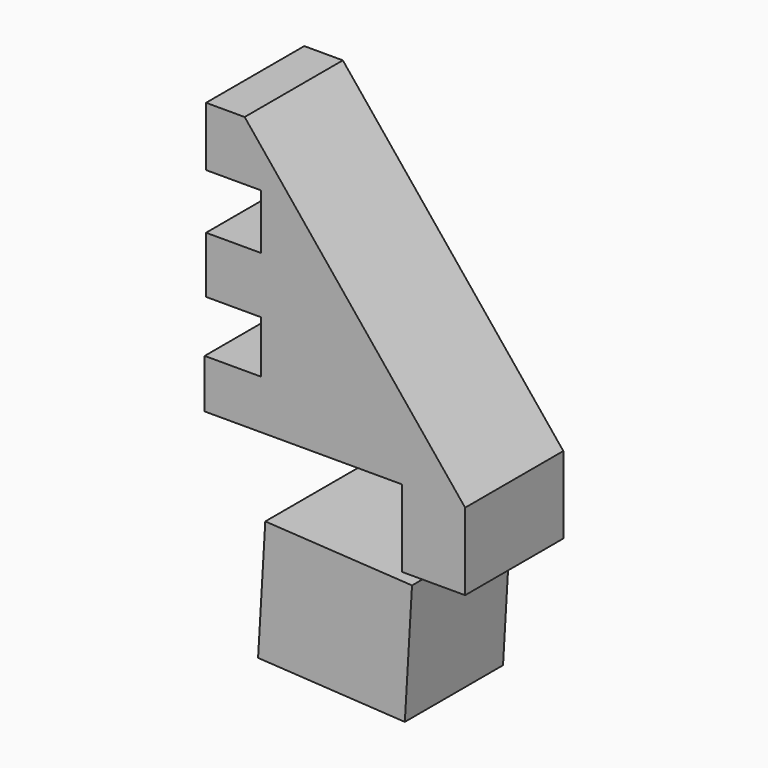
from build123d import *

# Parameters (mm, degrees)
F0_W     = 13.1069884534
F0_H     = 15.9477586227
F2_DEPTH = 25.4
F1_E23_W = 30.420306172
F1_E23_H = 25.4
F3_DEPTH = 25.4


with BuildPart() as f2:
    # F0 (on Front) → F2 (new body)
    with BuildSketch(Plane.XZ):
        Polygon((-3.4228879958, 56.3350282609), (-11.4096244797, 56.3350282609), (-11.4096244797, 44.0696775913), (0, 44.0696775913), (0, 32.6600521803), (-11.4096244797, 32.6600521803), (-11.4096244797, 20.9651887417), (0, 20.9651887417), (0, 10.1260431111), (-11.6948653013, 10.1260431111), (-11.6948653013, 0), (29.094543308, 0), (42.2015317614, 0), align=None)
        with Locations((35.6480375347, -7.9738793114)):
            Rectangle(F0_W, F0_H)
    extrude(amount=F2_DEPTH)


with BuildPart() as f3:
    # F1_E23 (on explicit) → F3 (new body)
    with BuildSketch(Plane(origin=(0.8463693679, 0, -15.9477586227), x_dir=(0.9982743725, 0, -0.0587220332), z_dir=(-0.0587220332, 0, -0.9982743725))):
        with Locations((15.210153086, 12.7)):
            Rectangle(F1_E23_W, F1_E23_H)
    extrude(amount=F3_DEPTH)


solid = Compound([f2.part, f3.part])
